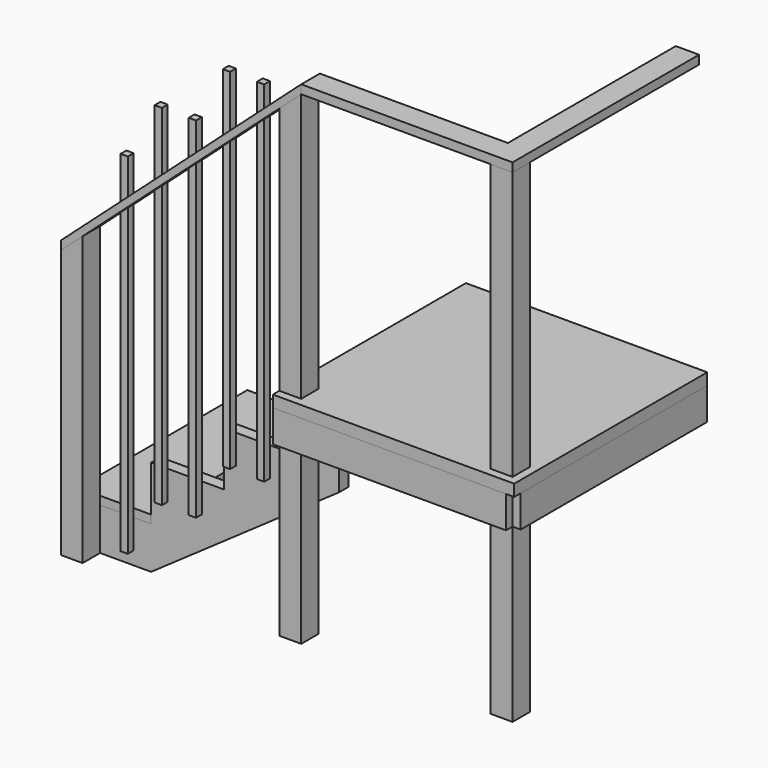
from build123d import *

# Parameters (mm, degrees)
F0_W      = 75
F0_H      = 75
F1_DEPTH  = 1690
F2_W      = 800
F2_H      = 110
F3_DEPTH  = 28
F4_W      = 800
F4_H      = 110
F5_DEPTH  = 28
F6_W      = 28
F6_H      = 110
F7_DEPTH  = 800
F8_W      = 28
F8_H      = 110
F9_DEPTH  = 697
F10_W     = 828
F10_H     = 828
F11_DEPTH = 40
F15_DEPTH = 40
F17_W     = 75
F17_H     = 75
F18_DEPTH = 1000
F20_DEPTH = 75
F22_DEPTH = 80
F24_DEPTH = 800.001
F25_W     = 25
F25_H     = 1200
F26_DEPTH = 25
F28_DEPTH = 30
F29_W     = 250
F29_H     = 725
F30_DEPTH = 28


with BuildPart() as f1:
    # F0 (on Top) → F1 (new body)
    with BuildSketch(Plane.XY):
        with Locations((37.5, 37.5)):
            Rectangle(F0_W, F0_H)
    extrude(amount=F1_DEPTH)

    # F23 (on face) → F24 (cut, through all)
    with BuildSketch(Plane.XZ):
        Polygon((0, 1690), (0, 1592.7272727273), (75, 1660), (75, 1690), align=None)
    extrude(amount=-F24_DEPTH, mode=Mode.SUBTRACT)


with BuildPart() as f1b:
    # F0 (on Top) → F1, piece 2 (new body)
    with BuildSketch(Plane.XY):
        with Locations((762.5, 37.5)):
            Rectangle(F0_W, F0_H)
    extrude(amount=F1_DEPTH)

    # F4 (on face) → F5 (join)
    with BuildSketch(Plane.YZ.offset(800)):
        with Locations((400, 645)):
            Rectangle(F4_W, F4_H)
    extrude(amount=F5_DEPTH)

    # F8 (on face) → F9 (join, through all)
    with BuildSketch(Plane(origin=(800, 0, 0), x_dir=(0, -1, 0), z_dir=(-1, 0, 0))):
        with Locations((-786, 645)):
            Rectangle(F8_W, F8_H)
    extrude(amount=F9_DEPTH)


with BuildPart() as f3:
    # F2 (on face) → F3 (new body)
    with BuildSketch(Plane.XZ):
        with Locations((400, 645)):
            Rectangle(F2_W, F2_H)
    extrude(amount=F3_DEPTH)


with BuildPart() as f7:
    # F6 (on face) → F7 (new body, through all)
    with BuildSketch(Plane(origin=(0, 0, 0), x_dir=(-1, 0, 0), z_dir=(0, 1, 0))):
        with Locations((-89, 645)):
            Rectangle(F6_W, F6_H)
    extrude(amount=F7_DEPTH)


with BuildPart() as f11:
    # F10 (on face) → F11 (new body)
    with BuildSketch(Plane.XY.offset(700)):
        with Locations((414, 386)):
            Rectangle(F10_W, F10_H)
    extrude(amount=F11_DEPTH)


with BuildPart() as f15:
    # F14 (on offset) → F15 (new body)
    with BuildSketch(Plane(origin=(0, 75, 0), x_dir=(-1, 0, 0), z_dir=(0, 1, 0))):
        Polygon((0, 700), (-145, 700), (-145, 450), (500, 0), (750, 0), (750, 145), (500, 145), (500, 330), (250, 330), (250, 515), (0, 515), align=None)
    extrude(amount=F15_DEPTH)


with BuildPart() as f16_1:
    # F16: instance of F15
    add(f15.part.mirror(Plane(origin=(37.5, 375, 845), x_dir=(-1, 0, 0), z_dir=(0, 1, 0))))


with BuildPart() as f15_1:
    add(f15.part)

    # F17 (on face) → F18 (join)
    with BuildSketch(Plane(origin=(0, 0, 0), x_dir=(1, 0, 0), z_dir=(0, 0, -1))):
        with Locations((-712.5, -37.5)):
            Rectangle(F17_W, F17_H)
    extrude(amount=-F18_DEPTH)

    # F19 (on face) → F20 (cut, through all)
    with BuildSketch(Plane.XZ):
        Polygon((-750, 1000), (-750, 920), (-675, 987.2727272727), (-675, 1000), align=None)
    extrude(amount=-F20_DEPTH, mode=Mode.SUBTRACT)


with BuildPart() as f22:
    # F21 (on face) → F22 (new body)
    with BuildSketch(Plane.XZ):
        Polygon((75, 1690), (-750, 950), (-750, 920), (75, 1660), align=None)
    extrude(amount=-F22_DEPTH)


with BuildPart() as f26:
    # F25 (on face) → F26 (new body)
    with BuildSketch(Plane.XZ.offset(-75)):
        with Locations((-338.5, 830)):
            Rectangle(F25_W, F25_H)
    extrude(amount=F26_DEPTH)


with BuildPart() as f26b:
    # F25 (on face) → F26, piece 2 (new body)
    with BuildSketch(Plane.XZ.offset(-75)):
        with Locations((-221.5, 1015)):
            Rectangle(F25_W, F25_H)
    extrude(amount=F26_DEPTH)


with BuildPart() as f26c:
    # F25 (on face) → F26, piece 3 (new body)
    with BuildSketch(Plane.XZ.offset(-75)):
        with Locations((-104.5, 1015)):
            Rectangle(F25_W, F25_H)
    extrude(amount=F26_DEPTH)


with BuildPart() as f26d:
    # F25 (on face) → F26, piece 4 (new body)
    with BuildSketch(Plane.XZ.offset(-75)):
        with Locations((-455.5, 830)):
            Rectangle(F25_W, F25_H)
    extrude(amount=F26_DEPTH)


with BuildPart() as f26e:
    # F25 (on face) → F26, piece 5 (new body)
    with BuildSketch(Plane.XZ.offset(-75)):
        with Locations((-572.5, 645)):
            Rectangle(F25_W, F25_H)
    extrude(amount=F26_DEPTH)


with BuildPart() as f28:
    # F27 (on face) → F28 (new body)
    with BuildSketch(Plane.XY.offset(1690)):
        Polygon((800, 800), (720, 800), (720, 80), (75, 80), (75, 0), (725, 0), (800, 0), align=None)
    extrude(amount=-F28_DEPTH)


with BuildPart() as f30:
    # F29 (on face) → F30 (new body)
    with BuildSketch(Plane.XY.offset(145)):
        with Locations((-625, 437.5)):
            Rectangle(F29_W, F29_H)
    extrude(amount=F30_DEPTH)


solid = Compound([f1.part, f1b.part, f3.part, f7.part, f11.part, f16_1.part, f15_1.part, f22.part, f26.part, f26b.part, f26c.part, f26d.part, f26e.part, f28.part, f30.part])
